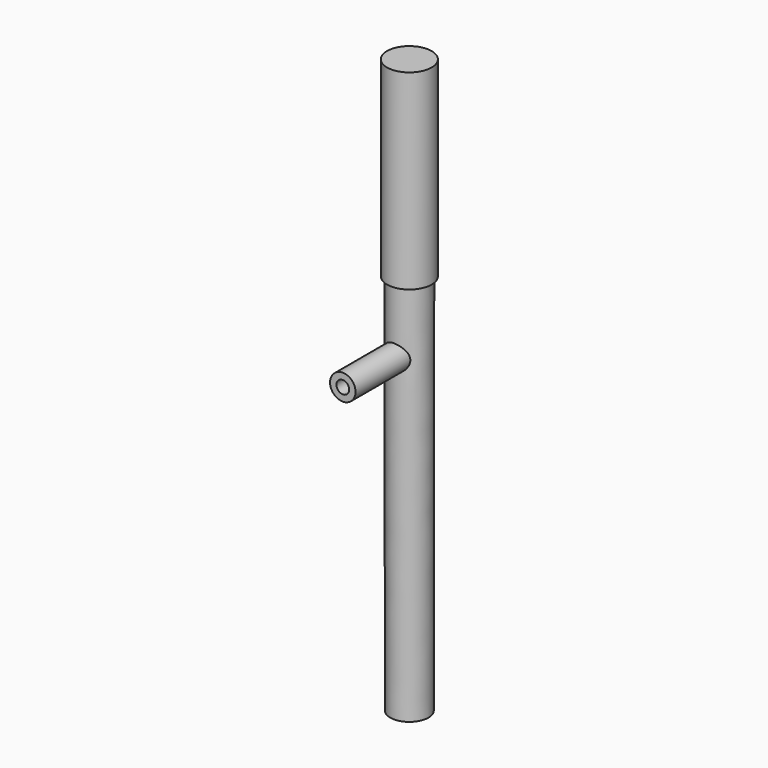
from build123d import *

# Parameters (mm, degrees)
F4_R     = 0.5
F5_REACH = 4.6934378881
F4_R_2   = 1
F7_DEPTH = 5


with BuildPart() as f1:
    # F0 (on Front) → F1 (revolve)
    with BuildSketch(Plane.XZ):
        with BuildLine():
            Line((-1.5291632199, 14.9999860381), (-1.5, -14.999999787))
            ThreePointArc((-1.5, -14.999999787), (-1, -14.499999787), (-0.5, -14.999999787))
            Line((-0.5, -14.999999787), (-0.5000000003, 10.500000213))
            Line((-0.5000000003, 10.500000213), (-3e-10, 10.500000213))
            Line((-3e-10, 10.500000213), (-3e-10, 30.000000213))
            Line((-3e-10, 30.000000213), (-1.7500000003, 30.000000213))
            Line((-1.7500000003, 30.000000213), (-1.7500000003, 14.9999860381))
            Line((-1.7500000003, 14.9999860381), (-1.5291632199, 14.9999860381))
        make_face()
    revolve(axis=Axis((-3e-10, 0, 7.500000213), (0, 0, -1)))

    f5_end = f1.faces().sort_by_distance((0.4999999994, 0, -2.249999787))[0]
    # F4 (on plane+point) → F5 (cut, up to a face of the model that its end follows)
    with BuildSketch(Plane.XZ.offset(1.5282243257)):
        with Locations((0, 10.000000213)):
            Circle(F4_R)
    f5_long = extrude(amount=-F5_REACH, mode=Mode.PRIVATE)
    add(split(f5_long, bisect_by=f5_end, keep=Keep.ALL, mode=Mode.PRIVATE).solids().sort_by_distance((0, -1.5282243257, 10.000000213))[0], mode=Mode.SUBTRACT)


with BuildPart() as f6:
    # F4 (on plane+point) → F6 (new body, up to the next surface of F1)
    with BuildSketch(Plane.XZ.offset(1.5282243257)):
        with Locations((0, 10.000000213)):
            Circle(F4_R_2)
        with Locations((0, 10.000000213)):
            Circle(F4_R, mode=Mode.SUBTRACT)
    extrude(until=Until.NEXT, target=f1.part, dir=(0, 1, 0))

    # F4 (on plane+point) → F7 (join)
    with BuildSketch(Plane.XZ.offset(1.5282243257)):
        with Locations((0, 10.000000213)):
            Circle(F4_R_2)
        with Locations((0, 10.000000213)):
            Circle(F4_R, mode=Mode.SUBTRACT)
    extrude(amount=F7_DEPTH)


solid = Compound([f1.part, f6.part])
